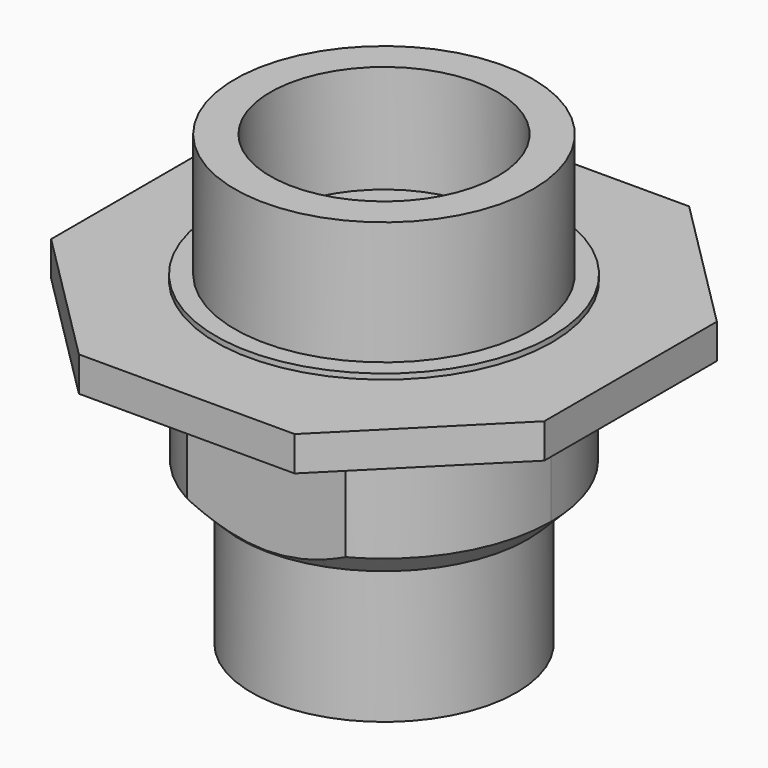
from build123d import *

# Parameters (mm, degrees)
F1_DEPTH    = 2.25
F2_R        = 10.9
F3_DEPTH    = 10.6
F5_DEPTH    = 9.5
F6_T2_ANGLE = 290.6956436441
F6_T4_ANGLE = 110.5630137602
F7_R        = 8.6
F8_DEPTH    = 10
F9_R        = 7.38
F10_DEPTH   = 7
F11_R       = 10.9
F11_R_2     = 9.6734059383
F12_DEPTH   = 8
F13_R       = 9.5
F14_DEPTH   = 1


# Not quite as in the source:
# - a fillet or chamfer that OpenCascade refuses, or shapes differently, is made with other operations: its cross-section is extruded or revolved along the edge and cut away or added


with BuildPart() as f1:
    # F0 (on Top) → F1 (new body)
    with BuildSketch(Plane.XY):
        Polygon((0, 9), (9, 0), (23, 0), (32, 9), (32, 23), (23, 32), (9, 32), (0, 23), align=None)
    extrude(amount=F1_DEPTH)

    # F2 (on Top) → F3 (join)
    with BuildSketch(Plane.XY):
        with Locations((16, 16)):
            Circle(F2_R)
    extrude(amount=F3_DEPTH)

    # F4 (on face) → F5 (join)
    with BuildSketch(Plane(origin=(0, 0, 0), x_dir=(1, 0, 0), z_dir=(0, 0, -1))):
        with BuildLine():
            ThreePointArc((10.8502427242, -6.45), (10.4390813008, -25.3165810908), (26.85, -16))
            ThreePointArc((26.85, -16), (25.3165810908, -10.4390813008), (21.1497572758, -6.45))
            Line((21.1497572758, -6.45), (10.8502427242, -6.45))
        make_face()
    extrude(amount=F5_DEPTH)

    # F6: chamfer of 1.5 on 2 edges, made by hand

    # F6_s1 → F6_t2 (revolve, cut)
    with BuildSketch(Plane(origin=(19.2912753227, 7.2878893438, 0), x_dir=(0, 0, 1), z_dir=(0.9354709038, 0.3534037184, 0))):
        with BuildLine():
            Line((-7.9575735931, 1.5793514401), (-9.5424264069, -0.0055013736))
            Line((-9.5424264069, -0.0055013736), (-9.5724264069, -0.0055013736))
            ThreePointArc((-9.5724264069, -0.0055013736), (-9.53, 0.7657118298), (-9.53, 1.5369250333))
            Line((-9.53, 1.5369250333), (-9.5, 1.5669250333))
            ThreePointArc((-9.5, 1.5669250333), (-8.7287867966, 1.5669250333), (-7.9575735931, 1.6093514401))
            Line((-7.9575735931, 1.6093514401), (-7.9575735931, 1.5793514401))
        make_face()
    revolve(axis=Axis((16, 16, -9.5), (0, 0, -1)), revolution_arc=F6_T2_ANGLE, mode=Mode.SUBTRACT)

    # F6_s3 → F6_t4 (revolve, cut)
    with BuildSketch(Plane.XZ.offset(-16)):
        with BuildLine():
            Line((26.8924264069, -7.9575735931), (25.3075735931, -9.5424264069))
            Line((25.3075735931, -9.5424264069), (25.3075735931, -9.5724264069))
            ThreePointArc((25.3075735931, -9.5724264069), (26.0787867966, -9.53), (26.85, -9.53))
            Line((26.85, -9.53), (26.88, -9.5))
            ThreePointArc((26.88, -9.5), (26.88, -8.7287867966), (26.9224264069, -7.9575735931))
            Line((26.9224264069, -7.9575735931), (26.8924264069, -7.9575735931))
        make_face()
    revolve(axis=Axis((16, 16, -9.5), (0, 0, -1)), revolution_arc=F6_T4_ANGLE, mode=Mode.SUBTRACT)

    # F7 (on face) → F8 (join)
    with BuildSketch(Plane(origin=(0, 0, -9.5), x_dir=(1, 0, 0), z_dir=(0, 0, -1))):
        with Locations((16, -16)):
            Circle(F7_R)
    extrude(amount=F8_DEPTH)

    # F9 (on face) → F10 (cut)
    with BuildSketch(Plane.XY.offset(10.6)):
        with Locations((16, 16)):
            Circle(F9_R)
    extrude(amount=-F10_DEPTH, mode=Mode.SUBTRACT)

    # F11 (on face) → F12 (cut)
    with BuildSketch(Plane.XY.offset(10.6)):
        with Locations((16, 16)):
            Circle(F11_R)
        with Locations((16, 16)):
            Circle(F11_R_2, mode=Mode.SUBTRACT)
    extrude(amount=-F12_DEPTH, mode=Mode.SUBTRACT)

    # F13 (on face) → F14 (cut)
    with BuildSketch(Plane(origin=(0, 0, -19.5), x_dir=(1, 0, 0), z_dir=(0, 0, -1))):
        with Locations((16, -16)):
            Circle(F13_R)
    extrude(amount=-F14_DEPTH, mode=Mode.SUBTRACT)


solid = f1.part
